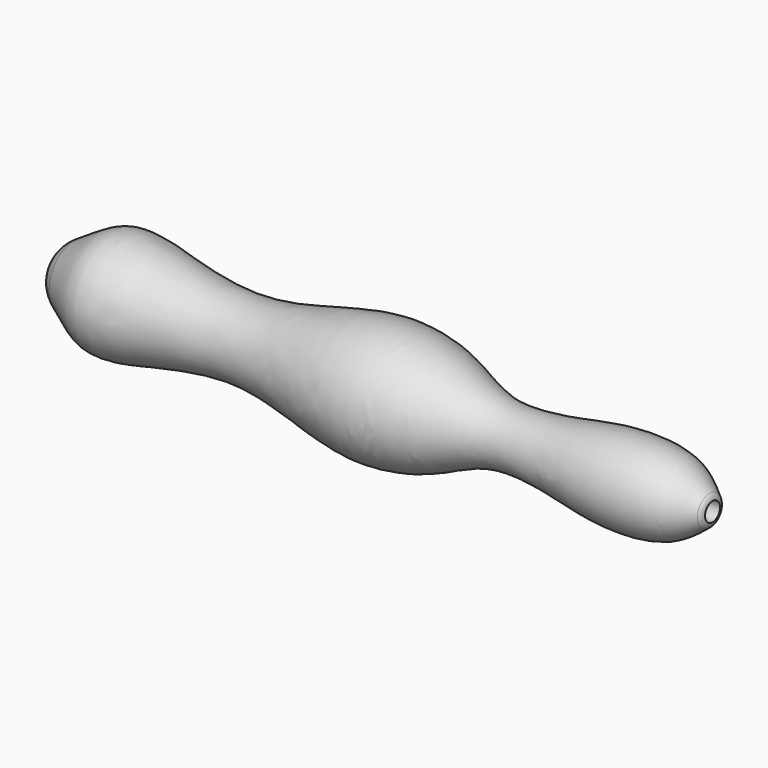
from build123d import *

# Parameters (mm, degrees)
F2_R     = 2
F3_DEPTH = 140.0010001


# Not quite as in the source:
# - a fillet or chamfer that OpenCascade refuses, or shapes differently, is made with other operations: its cross-section is extruded or revolved along the edge and cut away or added


with BuildPart() as f1:
    # F0 (on Top) → F1 (revolve)
    with BuildSketch(Plane.XY):
        with BuildLine():
            Line((0, 5), (0, 0))
            Line((0, 0), (140, 0))
            Line((140, 0), (140, 2.7142855423))
            add(Edge.make_bspline(
                [(0, 5), (4.9757928307, 6.8903925487), (10.237697674, 12.9335968557), (23.6587376595, 9.8681565944), (40.2335290349, 6.6148517626), (55.9344236845, 10.3648201497), (69.9820716554, 13.8213637044), (84.0708721521, 11.08852401), (95.0040113038, 4.316439134), (112.9408147187, 7.7663893472), (121.4997603993, 9.0367049085), (133.2708596303, 8.51780716), (137.8589455035, 4.4675047231), (140, 2.7142855423)],
                knots=[0, 0, 0, 0, 0.0894612415, 0.1774833365, 0.281696833, 0.3826889283, 0.4782971476, 0.5714614637, 0.6613001063, 0.7658299525, 0.8426077345, 0.9260031641, 1, 1, 1, 1], degree=3))
        make_face()
    revolve(axis=Axis((70, 0, 0), (1, 0, 0)))

    # F2 (on face) → F3 (cut, through all)
    with BuildSketch(Plane.YZ.offset(140)):
        Circle(F2_R)
    extrude(amount=-F3_DEPTH, mode=Mode.SUBTRACT)

    # F4: fillet of radius 7.62 on 1 edges, made by hand

    # F4_s1 → F4_t2 (revolve, cut)
    with BuildSketch(Plane.XY):
        with BuildLine():
            ThreePointArc((0, 2), (1.3103638059, 4.7185458275), (3.573309158, 6.7151987902))
            Line((3.573309158, 6.7151987902), (3.4971059638, 6.8471792175))
            ThreePointArc((3.4971059638, 6.8471792175), (1.7554490429, 5.9222679087), (-0.0541249607, 5.1424649032))
            Line((-0.0541249607, 5.1424649032), (-0.1524, 5))
            ThreePointArc((-0.1524, 5), (-0.1524, 3.5), (-0.1476693773, 2.0376764515))
            Line((-0.1476693773, 2.0376764515), (0, 2))
        make_face()
    revolve(axis=Axis((0, 0, 0), (1, 0, 0)), mode=Mode.SUBTRACT)

    # F5: fillet of radius 1.778 on 1 edges, made by hand

    # F5_s1 → F5_t2 (revolve, cut)
    with BuildSketch(Plane.XY):
        with BuildLine():
            ThreePointArc((140, 2), (139.8062268067, 2.6872174566), (139.3577242723, 3.2427904579))
            Line((139.3577242723, 3.2427904579), (139.3803449121, 3.270228028))
            ThreePointArc((139.3803449121, 3.270228028), (139.7012472414, 3.0057217978), (140.0225290745, 2.7417983466))
            Line((140.0225290745, 2.7417983466), (140.03556, 2.7142855423))
            ThreePointArc((140.03556, 2.7142855423), (140.03556, 2.3571427711), (140.0354661544, 2.0025817609))
            Line((140.0354661544, 2.0025817609), (140, 2))
        make_face()
    revolve(axis=Axis((140, 0, 0), (1, 0, 0)), mode=Mode.SUBTRACT)


solid = f1.part
